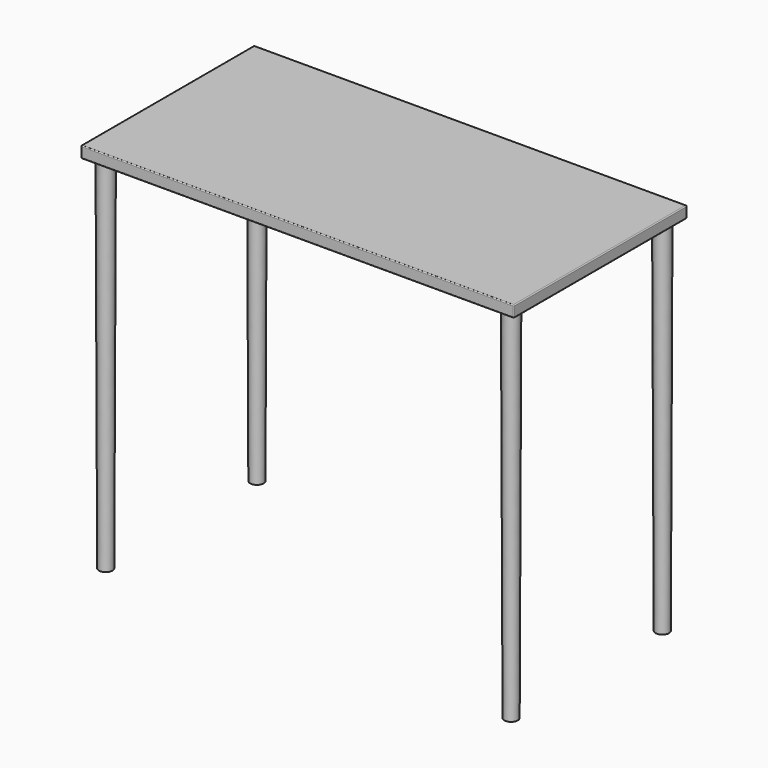
from build123d import *

# Parameters (mm, degrees)
F0_W     = 1200.15
F0_H     = 600.075
F1_DEPTH = 31.75
F2_R     = 2.54
F3_R     = 22.098
F4_DEPTH = 1003.3
F4_TAPER = 0.2
F5_SCALE = 0.05


with BuildPart() as f1:
    # F0 (on Top) → F1 (new body)
    with BuildSketch(Plane.XY):
        Rectangle(F0_W, F0_H)
    extrude(amount=F1_DEPTH)

    # F2
    f2_edges = [f1.edges().sort_by_distance(p)[0] for p in [
        (600.075, 300.0375, 15.875),
        (-600.075, 300.0375, 15.875),
        (0, 300.0375, 0),
        (0, 300.0375, 31.75),
        (-600.075, 0, 0),
        (0, -300.0375, 0),
        (600.075, 0, 0),
        (-600.075, 0, 31.75),
        (0, -300.0375, 31.75),
        (600.075, 0, 31.75),
        (-600.075, -300.0375, 15.875),
        (600.075, -300.0375, 15.875),
    ]]
    fillet(f2_edges, radius=F2_R)

    # F3 (on face) → F4 (join)
    with BuildSketch(Plane(origin=(0, 0, 0), x_dir=(1, 0, 0), z_dir=(0, 0, -1))):
        with Locations((-561.975, 261.9375)):
            Circle(F3_R)
        with Locations((561.975, 261.9375)):
            Circle(F3_R)
        with Locations((-561.975, -261.9375)):
            Circle(F3_R)
        with Locations((561.975, -261.9375)):
            Circle(F3_R)
    extrude(amount=F4_DEPTH, taper=F4_TAPER)


with BuildPart() as f1_1:
    # F5: moved
    add(f1.part.scale(F5_SCALE))


solid = f1_1.part
